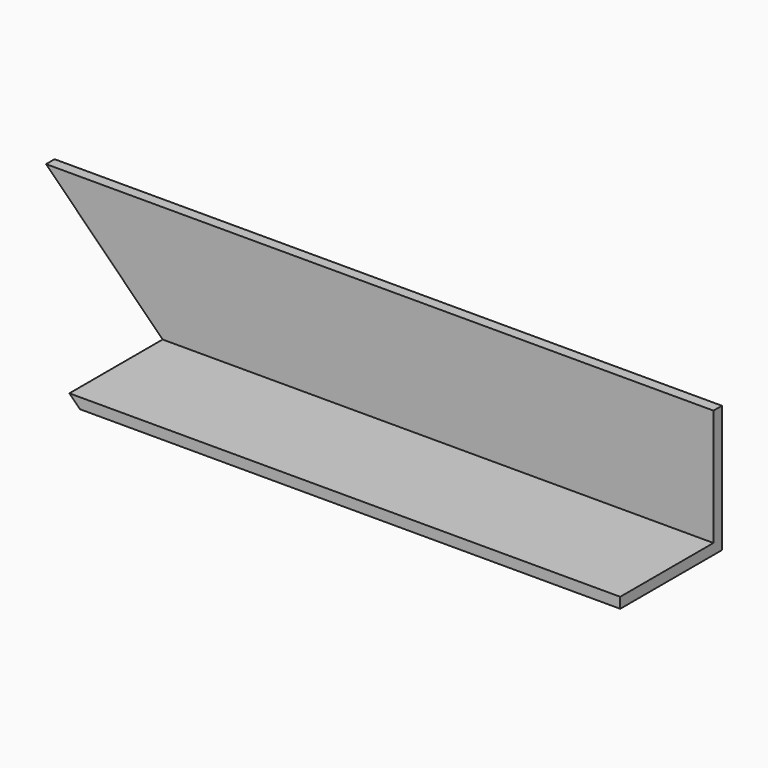
from build123d import *

# Parameters (mm, degrees)
F1_DEPTH = 6.35
F0_W     = 330.2
F0_H     = 6.35
F2_DEPTH = 76.2
F3_SIZE  = 6.34999


# Not quite as in the source:
# - a fillet or chamfer is up to 0.001 mm smaller than in the source, because OpenCascade refuses the exact size


with BuildPart() as f1:
    # F0 (on Front) → F1 (new body)
    with BuildSketch(Plane.XZ):
        Polygon((-339.7388204469, 69.3321084814), (-269.8888204469, -0.5178915186), (60.3111795531, -0.5178915186), (60.3111795531, 69.3321084814), align=None)
    extrude(amount=F1_DEPTH)

    # F0 (on Front) → F2 (join)
    with BuildSketch(Plane.XZ):
        with Locations((-104.7888204469, -3.6928915186)):
            Rectangle(F0_W, F0_H)
    extrude(amount=F2_DEPTH)

    # F3 (size 6.35 in the source; OpenCascade refuses exactly that, so slightly less here)
    f3_edges = [f1.edges().sort_by_distance(p)[0] for p in [
        (-269.88882, -38.1, -6.867892),
    ]]
    chamfer(f3_edges, length=F3_SIZE)


solid = f1.part
